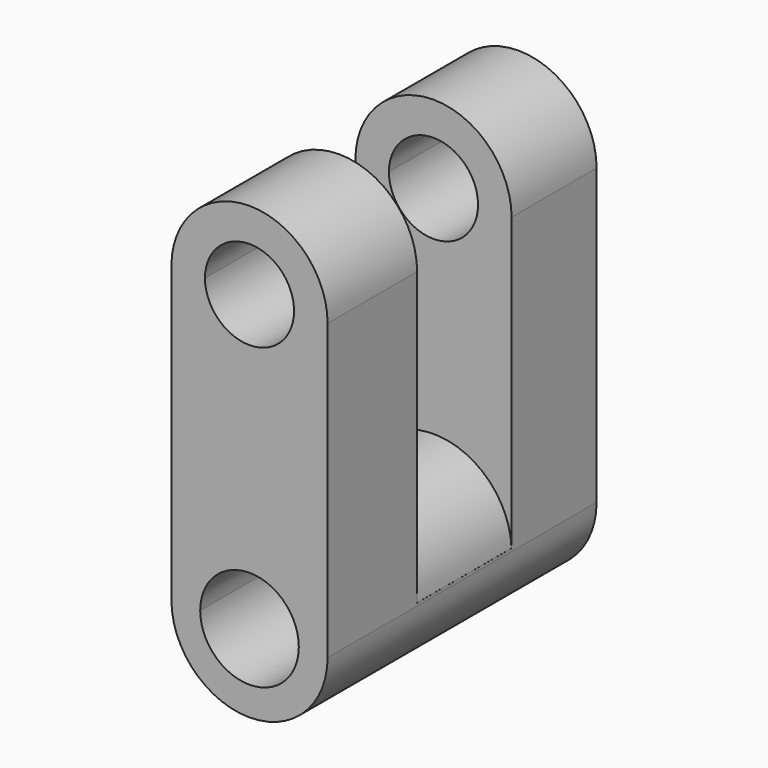
from build123d import *

# Parameters (mm, degrees)
F1_DEPTH      = 50.8
F1_DEPTH_BACK = 50.8
F2_W          = 18.690553
F2_H          = 120.086703
F3_DEPTH      = 152.4
F3_DEPTH_BACK = 152.4
F4_DEPTH      = 25.4
F4_DEPTH_BACK = 25.4


with BuildPart() as f1:
    # F0 (on Front) → F1 (new body, two sides)
    with BuildSketch(Plane.XZ) as f1_sk:
        with BuildLine():
            ThreePointArc((-23.595735, 44.451416), (0, 20.85568), (23.595735, 44.451416))
            Line((23.595735, 44.451416), (13.459783, 44.451416))
            ThreePointArc((13.459783, 44.451416), (0, 30.991633), (-13.459783, 44.451416))
            Line((-13.459783, 44.451416), (-23.595735, 44.451416))
        make_face()
        with BuildLine():
            Line((13.459783, 44.451416), (23.595735, 44.451416))
            ThreePointArc((23.595735, 44.451416), (0, 68.047151), (-23.595735, 44.451416))
            Line((-23.595735, 44.451416), (-13.459783, 44.451416))
            ThreePointArc((-13.459783, 44.451416), (0, 57.911198), (13.459783, 44.451416))
        make_face()
        with BuildLine():
            Line((23.595735, -44.451416), (23.595735, 44.451416))
            ThreePointArc((23.595735, 44.451416), (0, 20.85568), (-23.595735, 44.451416))
            Line((-23.595735, 44.451416), (-23.595735, -44.451416))
            ThreePointArc((-23.595735, -44.451416), (0, -20.85568), (23.595735, -44.451416))
        make_face()
        with BuildLine():
            ThreePointArc((-23.595735, -44.451416), (0, -68.047151), (23.595735, -44.451416))
            Line((23.595735, -44.451416), (14.896513, -44.451416))
            ThreePointArc((14.896513, -44.451416), (0, -59.347928), (-14.896513, -44.451416))
            Line((-14.896513, -44.451416), (-23.595735, -44.451416))
        make_face()
        with BuildLine():
            Line((14.896513, -44.451416), (23.595735, -44.451416))
            ThreePointArc((23.595735, -44.451416), (0, -20.85568), (-23.595735, -44.451416))
            Line((-23.595735, -44.451416), (-14.896513, -44.451416))
            ThreePointArc((-14.896513, -44.451416), (0, -29.554903), (14.896513, -44.451416))
        make_face()
    extrude(amount=F1_DEPTH)
    extrude(f1_sk.sketch, amount=-F1_DEPTH_BACK)

    # F2 (on face) → F3 (cut, two sides)
    with BuildSketch(Plane(origin=(-23.595735, 0, 0), x_dir=(0, -1, 0), z_dir=(-1, 0, 0))) as f3_sk:
        Polygon((0, 76.457053), (0, -43.62965), (16.988121, -43.62965), (16.988121, 76.525114), (0, 76.525114), align=None)
        with Locations((-9.345276, 16.413702)):
            Rectangle(F2_W, F2_H)
    extrude(amount=-F3_DEPTH, mode=Mode.SUBTRACT)
    extrude(f3_sk.sketch, amount=F3_DEPTH_BACK, mode=Mode.SUBTRACT)

    # F0 (on Front) → F4 (join, two sides)
    with BuildSketch(Plane.XZ) as f4_sk:
        with BuildLine():
            Line((14.896513, -44.451416), (23.595735, -44.451416))
            ThreePointArc((23.595735, -44.451416), (0, -20.85568), (-23.595735, -44.451416))
            Line((-23.595735, -44.451416), (-14.896513, -44.451416))
            ThreePointArc((-14.896513, -44.451416), (0, -29.554903), (14.896513, -44.451416))
        make_face()
    extrude(amount=F4_DEPTH)
    extrude(f4_sk.sketch, amount=-F4_DEPTH_BACK)


solid = f1.part
